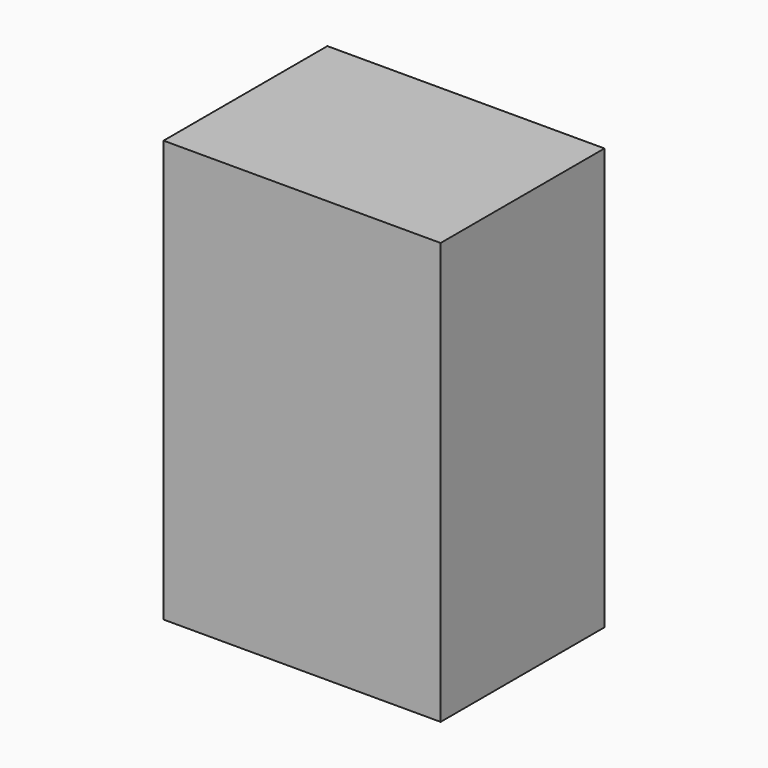
from build123d import *

# Parameters (mm, degrees)
F0_W     = 11.5
F0_H     = 17.5
F1_DEPTH = 8.5


# Not quite as in the source:
# - the program builds the solid bodies; features that only make, move or delete a surface that nothing else refers to are left out


with BuildPart() as f1:
    # F0 (on Front) → F1 (new body)
    with BuildSketch(Plane.XZ):
        Rectangle(F0_W, F0_H)
    extrude(amount=-F1_DEPTH)


solid = f1.part
